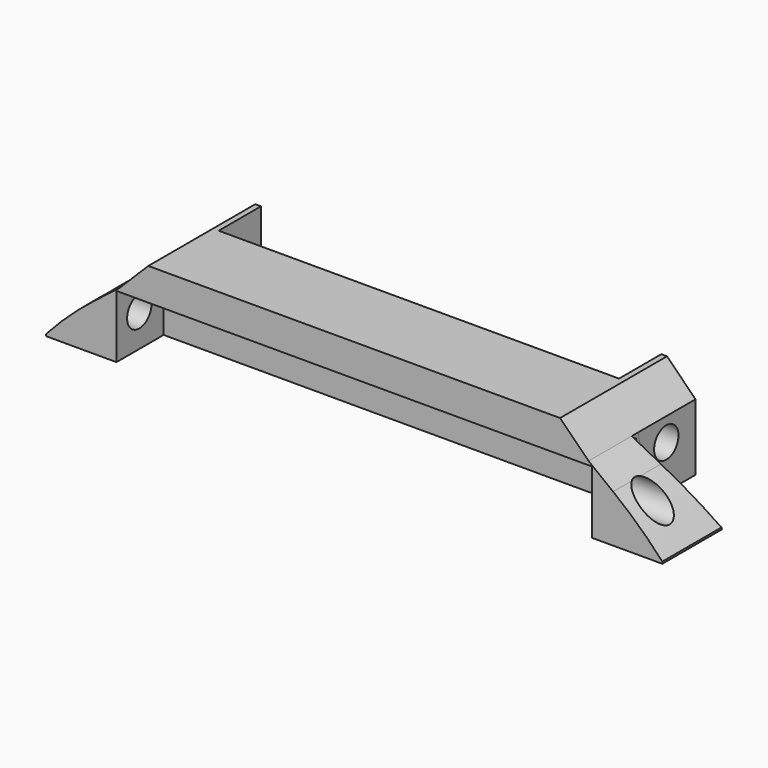
from build123d import *

# Parameters (mm, degrees)
F1_R           = 1.6
F2_DEPTH       = 33
F2_DEPTH_BACK  = 33
F4_DEPTH       = 62.0586978075
F8_W           = 6.3
F8_H           = 7
F9_DEPTH       = 25
F9_DEPTH_BACK  = 25
F10_R          = 1.6
F11_DEPTH      = 32.4035001
F11_DEPTH_BACK = 32.4035001
F13_DEPTH      = 3
F14_W          = 42.103
F14_H          = 3
F15_DEPTH      = 2
F16_SIZE       = 2.99999
F18_DEPTH      = 25


# Not quite as in the source:
# - a fillet or chamfer is up to 0.001 mm smaller than in the source, because OpenCascade refuses the exact size
# - a pattern or mirror of a feature is missing from the dataset's text; its kind, count and spacing are read off the source's solid


with BuildPart() as f2:
    # F1 (on offset) → F2 (new body, two sides)
    with BuildSketch(Plane.YZ.offset(-40)) as f2_sk:
        with BuildLine():
            Line((-55.5576978075, 47), (-62.0576978075, 47))
            Line((-62.0576978075, 47), (-62.0576978075, 40))
            Line((-62.0576978075, 40), (-53.0576978075, 40))
            ThreePointArc((-53.0576978075, 40), (-53.9183376958, 41.7448320543), (-54.7576978075, 43.5))
            ThreePointArc((-54.7576978075, 43.5), (-55.1675152463, 45.247756014), (-55.5576978075, 47))
        make_face()
        with Locations((-59.0576978075, 43.5)):
            Circle(F1_R, mode=Mode.SUBTRACT)
    extrude(amount=F2_DEPTH)
    extrude(f2_sk.sketch, amount=-F2_DEPTH_BACK)

    # F3 (on Front) → F4 (cut, through all)
    with BuildSketch(Plane.XZ):
        with BuildLine():
            ThreePointArc((-72.4025, 40.2057909187), (-69.9229908245, 42.7170557867), (-67.2317861301, 45))
            Line((-67.2317861301, 45), (-64.6515, 47))
            Line((-64.6515, 47), (-77.5247141719, 47))
            Line((-77.5247141719, 47), (-77.5247141719, 39.4350364804))
            Line((-77.5247141719, 39.4350364804), (-72.4025, 39.4350364804))
            Line((-72.4025, 39.4350364804), (-72.4025, 40.2057909187))
        make_face()
        with BuildLine():
            Line((-7.5975, 40.2057909187), (-7.5975, 39.4350364804))
            Line((-7.5975, 39.4350364804), (-2.4752858281, 39.4350364804))
            Line((-2.4752858281, 39.4350364804), (-2.4752858281, 47))
            Line((-2.4752858281, 47), (-15.3485, 47))
            Line((-15.3485, 47), (-12.7682138699, 45))
            ThreePointArc((-12.7682138699, 45), (-10.0770091755, 42.7170557867), (-7.5975, 40.2057909187))
        make_face()
    extrude(amount=F4_DEPTH, mode=Mode.SUBTRACT)

    # F6 (on offset) → F7 (join, up to the next surface of F2)
    with BuildSketch(Plane.XZ.offset(48)):
        Polygon((-64.6515, 47), (-64.6515, 44.9052631579), (-64.6515, 40), (-61.0515, 40), (-61.0515, 44.9052631579), (-61.0515, 47), align=None)
    f7 = extrude(until=Until.NEXT)

    # F7_copies: F7 across plane
    add(f7.mirror(Plane(origin=(-40.000004, 0, 3e-06), x_dir=(0, 0, 1), z_dir=(1, 0, 0))))

    # F8 (on offset) → F9 (cut, two sides)
    with BuildSketch(Plane.YZ.offset(-40)) as f9_sk:
        with Locations((-59.0076978075, 43.1)):
            Rectangle(F8_W, F8_H)
    extrude(amount=-F9_DEPTH, mode=Mode.SUBTRACT)
    extrude(f9_sk.sketch, amount=F9_DEPTH_BACK, mode=Mode.SUBTRACT)

    # F10 (on offset) → F11 (cut, two sides)
    with BuildSketch(Plane.YZ.offset(-40)) as f11_sk:
        with Locations((-51.845, 44.56195746)):
            Circle(F10_R)
    extrude(amount=-F11_DEPTH, mode=Mode.SUBTRACT)
    extrude(f11_sk.sketch, amount=F11_DEPTH_BACK, mode=Mode.SUBTRACT)

    # F12 (on face) → F13 (join)
    with BuildSketch(Plane.XY.offset(47)):
        Polygon((-64.6515, -48.0000000008), (-64.6515, -55.5576978083), (-64.6515, -62.0576978075), (-15.3485, -62.0576978075), (-15.3485, -55.5576978075), (-15.3485, -48.0000000007), (-18.9485, -48), (-18.9485, -55.5576978084), (-61.0515, -55.5576978075), (-61.0515, -48.0000000007), align=None)
    extrude(amount=F13_DEPTH)

    # F14 (on face) → F15 (join)
    with BuildSketch(Plane(origin=(0, -55.5576978075, 0), x_dir=(-1, 0, 0), z_dir=(0, 1, 0))):
        with Locations((40, 48.5)):
            Rectangle(F14_W, F14_H)
    extrude(amount=F15_DEPTH)

    # F16 (size 3 in the source; OpenCascade refuses exactly that, so slightly less here)
    f16_edges = [f2.edges().sort_by_distance(p)[0] for p in [
        (-64.6515, -55.028849, 50),
        (-15.3485, -55.028849, 50),
    ]]
    chamfer(f16_edges, length=F16_SIZE)

    # F17 (on face) → F18 (cut)
    with BuildSketch(Plane(origin=(-64.6515, 0, 0), x_dir=(0, -1, 0), z_dir=(-1, 0, 0))):
        Polygon((56.3939474523, 47), (55.5576978075, 47), (53.0576978075, 40), (54.2201250791, 40), align=None)
    f18 = extrude(amount=F18_DEPTH, mode=Mode.SUBTRACT)

    # F18_copies: F18 across plane
    add(f18.mirror(Plane(origin=(-40, 0, 0), x_dir=(0, 0, 1), z_dir=(1, 0, 0))), mode=Mode.SUBTRACT)


solid = f2.part
